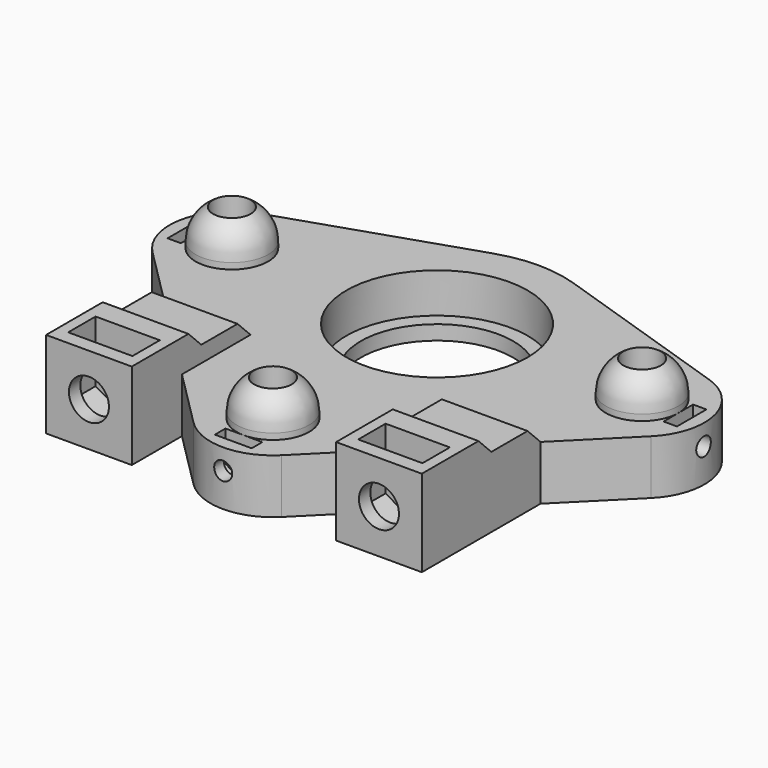
from build123d import *

# Parameters (mm, degrees)
F0_R          = 3.302
F0_R_2        = 15.875
F1_DEPTH      = 9.525
F0_R_3        = 13.335
F2_DEPTH      = 2.54
F5_DEPTH      = 8.636
F6_T1_DEPTH   = 2.3368
F6_T3_DEPTH   = 2.3368
F6_T5_DEPTH   = 2.3368
F3_R          = 6.35
F3_R_2        = 3.302
F7_DEPTH      = 6.35
F11_R         = 1.5875
F12_DEPTH     = 6.35
F9_R          = 1.5875
F13_DEPTH     = 6.35
F10_R         = 1.5875
F14_DEPTH     = 8.382
F16_DEPTH     = 5.6642
F15_W         = 15.0114
F15_H         = 10.748598603
F17_DEPTH     = 2.8448
F18_T4_DEPTH  = 29.6432475283
F18_T9_DEPTH  = 29.6432475283
F18_T14_DEPTH = 29.6432475283
F18_T19_DEPTH = 29.6432475283
F19_W         = 11.2522
F19_H         = 5.9944
F20_DEPTH     = 13.9954
F21_T1_DEPTH  = 20.5629100612
F22_T1_DEPTH  = 20.5167471751
F23_R         = 3.5052
F24_R         = 3.5052
F25_DEPTH     = 7.62


# Not quite as in the source:
# - a fillet or chamfer that OpenCascade refuses, or shapes differently, is made with other operations: its cross-section is extruded or revolved along the edge and cut away or added
# - a feature names something its author has since deleted; it is built from what else it names


with BuildPart() as f1:
    # F0 (on Top) → F1 (new body)
    with BuildSketch(Plane.XY):
        with BuildLine():
            Line((39.3578503288, 46.2881387371), (6.9933568382, 57.0169901512))
            ThreePointArc((6.9933568382, 57.0169901512), (0, 58.145934), (-6.9933568382, 57.0169901512))
            Line((-6.9933568382, 57.0169901512), (-39.3578503288, 46.2881387371))
            ThreePointArc((-39.3578503288, 46.2881387371), (-46.548869386, 38.4390523526), (-43.6441157783, 28.1978942818))
            Line((-43.6441157783, 28.1978942818), (-32.9057, 17.459532603))
            Line((-32.9057, 17.459532603), (-32.9057, -8.529066))
            Line((-32.9057, -8.529066), (-17.8943, -8.529066))
            Line((-17.8943, -8.529066), (-17.8943, 2.4482082294))
            Line((-17.8943, 2.4482082294), (-7.72300081, -7.7230397182))
            ThreePointArc((-7.72300081, -7.7230397182), (0, -10.922), (7.72300081, -7.7230397182))
            Line((7.72300081, -7.7230397182), (17.8943, 2.4482082294))
            Line((17.8943, 2.4482082294), (17.8943, -8.529066))
            Line((17.8943, -8.529066), (32.9057, -8.529066))
            Line((32.9057, -8.529066), (32.9057, 17.459532603))
            Line((32.9057, 17.459532603), (43.6441157783, 28.1978942818))
            ThreePointArc((43.6441157783, 28.1978942818), (46.548869386, 38.4390523526), (39.3578503288, 46.2881387371))
        make_face()
        Circle(F0_R, mode=Mode.SUBTRACT)
        with Locations((-35.9211149683, 35.920934)):
            Circle(F0_R, mode=Mode.SUBTRACT)
        with Locations((0, 35.920934)):
            Circle(F0_R_2, mode=Mode.SUBTRACT)
        with Locations((35.9211149683, 35.920934)):
            Circle(F0_R, mode=Mode.SUBTRACT)
    extrude(amount=F1_DEPTH)

    # F0 (on Top) → F2 (join)
    with BuildSketch(Plane.XY):
        with Locations((0, 35.920934)):
            Circle(F0_R_2)
        with Locations((0, 35.920934)):
            Circle(F0_R_3, mode=Mode.SUBTRACT)
    extrude(amount=F2_DEPTH)

    # F4 (on face) → F5 (cut)
    with BuildSketch(Plane.XY.offset(9.525)):
        Polygon((-42.2711149683, 32.695134), (-42.2711149683, 35.920934), (-42.2711149683, 39.146734), (-44.6079149683, 39.146734), (-44.6079149683, 32.695134), align=None)
        Polygon((42.2711149683, 39.146734), (42.2711149683, 35.920934), (42.2711149683, 32.695134), (44.6079149683, 32.695134), (44.6079149683, 39.146734), align=None)
        Polygon((3.2258, -6.35), (0, -6.35), (-3.2258, -6.35), (-3.2258, -8.6868), (3.2258, -8.6868), align=None)
    extrude(amount=-F5_DEPTH, mode=Mode.SUBTRACT)

    # F6: chamfer of 3.175 x 5.499261314 on 6 edges, made by hand

    # F6_s2 → F6_t1 (join)
    with BuildSketch(Plane.YZ.offset(-44.6079149683)):
        Polygon((39.146734, 4.064), (33.647472686, 0.889), (39.146734, 0.889), align=None)
        Polygon((32.695134, 4.064), (38.194395314, 0.889), (32.695134, 0.889), align=None)
    extrude(amount=F6_T1_DEPTH)

    # F6_s4 → F6_t3 (join)
    with BuildSketch(Plane.XZ.offset(6.35)):
        Polygon((3.2258, 4.064), (-2.273461314, 0.889), (3.2258, 0.889), align=None)
        Polygon((-3.2258, 4.064), (2.273461314, 0.889), (-3.2258, 0.889), align=None)
    extrude(amount=F6_T3_DEPTH)

    # F6_s6 → F6_t5 (join)
    with BuildSketch(Plane.YZ.offset(42.2711149683)):
        Polygon((39.146734, 4.064), (33.647472686, 0.889), (39.146734, 0.889), align=None)
        Polygon((32.695134, 4.064), (38.194395314, 0.889), (32.695134, 0.889), align=None)
    extrude(amount=F6_T5_DEPTH)

    # F3 (on face) → F7 (join)
    with BuildSketch(Plane.XY.offset(9.525)):
        with Locations((-35.9211149683, 35.920934)):
            Circle(F3_R)
        with Locations((-35.9211149683, 35.920934)):
            Circle(F3_R_2, mode=Mode.SUBTRACT)
        Circle(F3_R)
        Circle(F3_R_2, mode=Mode.SUBTRACT)
        with Locations((35.9211149683, 35.920934)):
            Circle(F3_R)
        with Locations((35.9211149683, 35.920934)):
            Circle(F3_R_2, mode=Mode.SUBTRACT)
    extrude(amount=F7_DEPTH)

    # F8: fillet of radius 6.096 on 3 edges, made by hand

    # F8_s1 → F8_t2 (revolve, cut)
    with BuildSketch(Plane.XZ.offset(-35.920934)):
        with BuildLine():
            ThreePointArc((-29.5711149683, 10.5957091385), (-30.3878241069, 13.6437091385), (-32.6191149683, 15.875))
            Line((-32.6191149683, 15.875), (-29.5711149683, 15.875))
            Line((-29.5711149683, 15.875), (-29.5711149683, 10.5957091385))
        make_face()
    revolve(axis=Axis((-35.9211149683, 35.920934, 15.875), (0, 0, 1)), mode=Mode.SUBTRACT)

    # F8_s3 → F8_t4 (revolve, cut)
    with BuildSketch(Plane.XZ.offset(-35.920934)):
        with BuildLine():
            ThreePointArc((42.2711149683, 10.5957091385), (41.4544058298, 13.6437091385), (39.2231149683, 15.875))
            Line((39.2231149683, 15.875), (42.2711149683, 15.875))
            Line((42.2711149683, 15.875), (42.2711149683, 10.5957091385))
        make_face()
    revolve(axis=Axis((35.9211149683, 35.920934, 15.875), (0, 0, 1)), mode=Mode.SUBTRACT)

    # F8_s5 → F8_t6 (revolve, cut)
    with BuildSketch(Plane.XZ):
        with BuildLine():
            ThreePointArc((6.35, 10.5957091385), (5.5332908615, 13.6437091385), (3.302, 15.875))
            Line((3.302, 15.875), (6.35, 15.875))
            Line((6.35, 15.875), (6.35, 10.5957091385))
        make_face()
    revolve(axis=Axis((0, 0, 15.875), (0, 0, 1)), mode=Mode.SUBTRACT)

    # F11 (on face) → F12 (cut, symmetric)
    with BuildSketch(Plane(origin=(44.6079149683, 0, 0), x_dir=(0, -1, 0), z_dir=(-1, 0, 0))):
        with Locations((-35.8627085169, 5.8928)):
            Circle(F11_R)
    extrude(amount=F12_DEPTH, both=True, mode=Mode.SUBTRACT)

    # F9 (on face) → F13 (cut, symmetric)
    with BuildSketch(Plane.YZ.offset(-44.6079149683)):
        with Locations((35.8627085169, 5.8928)):
            Circle(F9_R)
    extrude(amount=F13_DEPTH, both=True, mode=Mode.SUBTRACT)

    # F10 (on face) → F14 (cut, symmetric)
    with BuildSketch(Plane(origin=(0, -8.6868, 0), x_dir=(-1, 0, 0), z_dir=(0, 1, 0))):
        with Locations((0.0582254831, 5.8928)):
            Circle(F10_R)
    extrude(amount=F14_DEPTH, both=True, mode=Mode.SUBTRACT)

    # F15 (on face) → F16 (join)
    with BuildSketch(Plane.XY.offset(9.525)):
        Polygon((17.8943, 6.710934), (17.8943, 2.4482082294), (17.8943, -8.529066), (32.9057, -8.529066), (32.9057, 6.710934), align=None)
        Polygon((-32.9057, -8.529066), (-17.8943, -8.529066), (-17.8943, 2.4482082294), (-17.8943, 6.710934), (-32.9057, 6.710934), align=None)
    extrude(amount=F16_DEPTH)

    # F15 (on face) → F17 (join)
    with BuildSketch(Plane.XY.offset(9.525)):
        with Locations((-25.4, 12.0852333015)):
            Rectangle(F15_W, F15_H)
        with Locations((25.4, 12.0852333015)):
            Rectangle(F15_W, F15_H)
    extrude(amount=F17_DEPTH)

    # F18: chamfer of 2.8448 on 4 edges, made by hand


with BuildPart() as f18_tool2:
    # F18_s3 → F18_t4 (new body)
    with BuildSketch(Plane.YZ.offset(-10.5783762358)):
        Polygon((14.614732603, 12.3698), (17.459532603, 9.525), (17.459532603, 12.3698), align=None)
    extrude(amount=-F18_T4_DEPTH)

    split(bisect_by=Plane.XY.offset(9.525), keep=Keep.TOP)


with BuildPart() as f1_1:
    add(f1.part)

    # F18_t1: cut F18_tool2
    add(f18_tool2.part, mode=Mode.SUBTRACT)


with BuildPart() as f18_tool7:
    # F18_s8 → F18_t9 (new body)
    with BuildSketch(Plane.YZ.offset(40.2216237642)):
        Polygon((17.459532603, 9.525), (14.614732603, 12.3698), (17.459532603, 12.3698), align=None)
    extrude(amount=-F18_T9_DEPTH)

    split(bisect_by=Plane.XY.offset(9.525), keep=Keep.TOP)


with BuildPart() as f1_2:
    add(f1_1.part)

    # F18_t6: cut F18_tool7
    add(f18_tool7.part, mode=Mode.SUBTRACT)


with BuildPart() as f18_tool12:
    # F18_s13 → F18_t14 (new body)
    with BuildSketch(Plane.YZ.offset(-10.5783762358)):
        Polygon((6.710934, 12.3444), (3.866134, 15.1892), (6.710934, 15.1892), align=None)
    extrude(amount=-F18_T14_DEPTH)

    split(bisect_by=Plane.XY.offset(12.3698), keep=Keep.TOP)


with BuildPart() as f1_3:
    add(f1_2.part)

    # F18_t11: cut F18_tool12
    add(f18_tool12.part, mode=Mode.SUBTRACT)


with BuildPart() as f18_tool17:
    # F18_s18 → F18_t19 (new body)
    with BuildSketch(Plane.YZ.offset(40.2216237642)):
        Polygon((6.710934, 12.3444), (3.866134, 15.1892), (6.710934, 15.1892), align=None)
    extrude(amount=-F18_T19_DEPTH)

    split(bisect_by=Plane.XY.offset(12.3698), keep=Keep.TOP)


with BuildPart() as f1_4:
    add(f1_3.part)

    # F18_t16: cut F18_tool17
    add(f18_tool17.part, mode=Mode.SUBTRACT)

    # F19 (on face) → F20 (cut)
    with BuildSketch(Plane.XY.offset(15.1892)):
        with Locations((-25.4, -3.042666)):
            Rectangle(F19_W, F19_H)
        with Locations((25.4, -3.042666)):
            Rectangle(F19_W, F19_H)
    extrude(amount=-F20_DEPTH, mode=Mode.SUBTRACT)

    # F21: chamfer of 3.2512 x 5.6312435856 on 3 edges, made by hand

    # F21_s2 → F21_t1 (join)
    with BuildSketch(Plane.XZ.offset(-14.5230440612)):
        Polygon((-19.7739, 4.445), (-25.4051435856, 1.1938), (-19.7739, 1.1938), align=None)
        Polygon((-31.0261, 4.445), (-25.3948564144, 1.1938), (-31.0261, 1.1938), align=None)
        Polygon((31.0261, 4.445), (25.3948564144, 1.1938), (31.0261, 1.1938), align=None)
    extrude(amount=F21_T1_DEPTH)

    # F22: chamfer of 5.6134 x 3.2408980011 on 1 edges, made by hand

    # F22_s2 → F22_t1 (join)
    with BuildSketch(Plane.XZ.offset(-14.4768811751)):
        Polygon((19.7739, 4.4346980011), (25.3873, 1.1938), (19.7739, 1.1938), align=None)
    extrude(amount=F22_T1_DEPTH)

    # F23 (on face) + F24 (on face) → F25 (cut, symmetric)
    with BuildSketch(Plane(origin=(0, -6.039866, 0), x_dir=(-1, 0, 0), z_dir=(0, 1, 0))):
        with Locations((25.4, 7.6932303495)):
            Circle(F23_R)
    with BuildSketch(Plane(origin=(0, -6.039866, 0), x_dir=(-1, 0, 0), z_dir=(0, 1, 0))):
        with Locations((-25.3948564144, 7.6962)):
            Circle(F24_R)
    extrude(amount=F25_DEPTH, both=True, mode=Mode.SUBTRACT)


solid = f1_4.part
